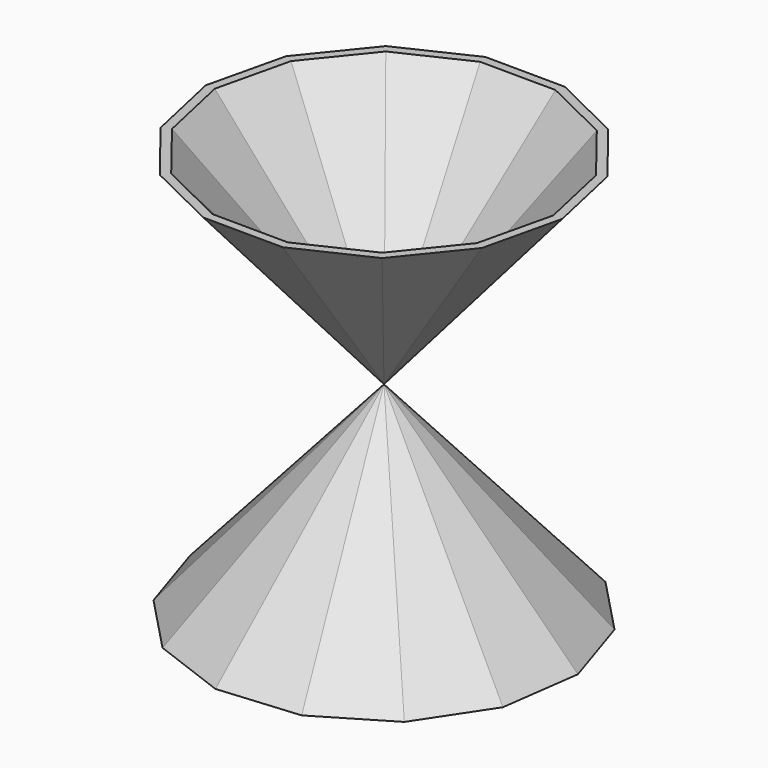
from build123d import *

# Parameters (mm, degrees)
F3_T = -2.5
F7_T = -2.5


# Not quite as in the source:
# - the program builds the solid bodies; features that only make, move or delete a surface that nothing else refers to are left out


with BuildPart() as f2:
    # F1 (on offset) → F2 section 0
    with BuildSketch(Plane.XY.offset(75.5), mode=Mode.PRIVATE) as f2_s0:
        Polygon((-40.9395454607, 52.0532105827), (-59.4702975669, 29.1353191471), (-66.2222278846, 0.4468204332), (-59.8580338074, -28.3301765474), (-41.6382220241, -51.496034616), (-15.1714497096, -64.4624714714), (14.3002142855, -64.6613252717), (40.9395454607, -52.0532105827), (59.4702975669, -29.1353191471), (66.2222278846, -0.4468204332), (59.8580338074, 28.3301765474), (41.6382220241, 51.496034616), (15.1714497096, 64.4624714714), (-14.3002142855, 64.6613252717), align=None)
    loft([f2_s0.sketch, Vertex(0, 0, 0)])

    # F3
    f3_openings = [f2.faces().sort_by_distance(p)[0] for p in [
        (0, 0, 75.5),
    ]]
    offset(amount=F3_T, openings=f3_openings)


with BuildPart() as f6:
    # F5 (on offset) → F6 section 0
    with BuildSketch(Plane.XY.offset(-75), mode=Mode.PRIVATE) as f6_s0:
        Polygon((-57.6491183851, -34.3802773844), (-37.0230176236, -55.9885746349), (-9.0640541642, -66.5076480243), (20.6901563858, -63.8540660596), (46.3464277154, -48.5534031931), (62.8232206344, -23.6361433558), (66.8571042305, 5.9625445514), (57.6491183851, 34.3802773844), (37.0230176236, 55.9885746349), (9.0640541642, 66.5076480243), (-20.6901563858, 63.8540660596), (-46.3464277154, 48.5534031931), (-62.8232206344, 23.6361433558), (-66.8571042305, -5.9625445514), align=None)
    loft([f6_s0.sketch, Vertex(0, 0, 0)])

    # F7
    f7_openings = [f6.faces().sort_by_distance(p)[0] for p in [
        (0, 0, -75),
    ]]
    offset(amount=F7_T, openings=f7_openings)


solid = Compound([f2.part, f6.part])
